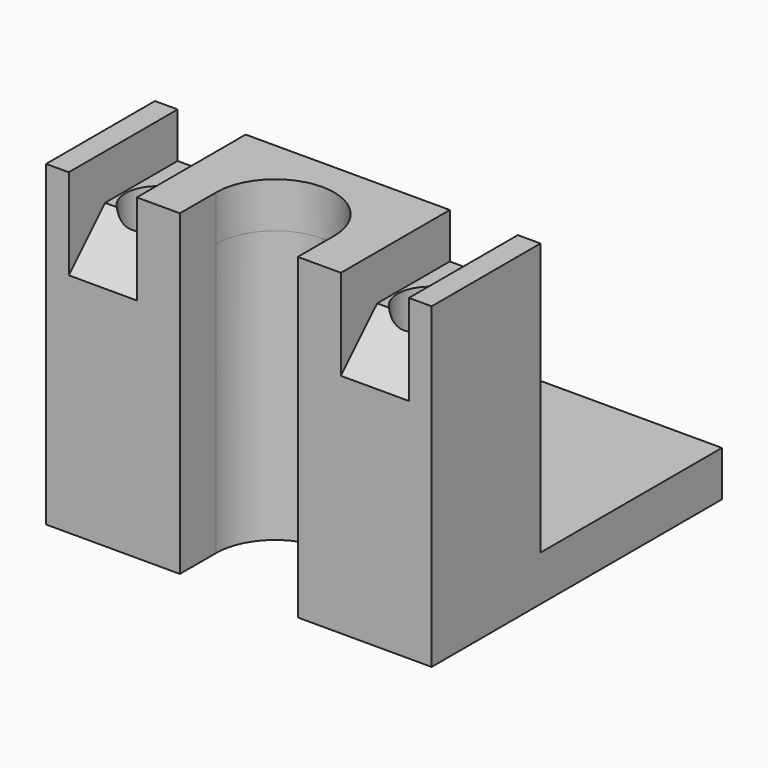
from build123d import *

# Parameters (mm, degrees)
F1_DEPTH    = 12
F0_W        = 8.5
F0_H        = 10
F2_DEPTH    = 2
F4_D        = 2.8
F6_W        = 1
F6_H        = 6
F7_DEPTH    = 2
F8_T1_DEPTH = 3
F8_T3_DEPTH = 3


# Not quite as in the source:
# - a fillet or chamfer that OpenCascade refuses, or shapes differently, is made with other operations: its cross-section is extruded or revolved along the edge and cut away or added


with BuildPart() as f1:
    # F0 (on Top) → F1 (new body)
    with BuildSketch(Plane.XY):
        with BuildLine():
            Line((0, 2), (0, 0))
            Line((0, 0), (5.9, 0))
            Line((5.9, 0), (5.9, 6))
            Line((5.9, 6), (-2.6, 6))
            Line((-2.6, 6), (-2.6, 4.6))
            ThreePointArc((-2.6, 4.6), (-0.7615223689, 3.8384776311), (0, 2))
        make_face()
    extrude(amount=F1_DEPTH)

    # F0 (on Top) → F2 (join)
    with BuildSketch(Plane.XY):
        with Locations((1.65, 11)):
            Rectangle(F0_W, F0_H)
    extrude(amount=F2_DEPTH)

    # F4 (through all)
    with Locations(Plane.XY.offset(12)):
        with Locations((3.4, 3)):
            Hole(F4_D / 2)

    # F5: F1 across face


with BuildPart() as f1_1:
    add(f1.part)
    add(f1.part.mirror(Plane(origin=(-2.6, 8.397826087, 3.2826086957), x_dir=(0, -1, 0), z_dir=(-1, 0, 0))))

    # F6 (on face) → F7 (join)
    with BuildSketch(Plane.XY.offset(12)):
        with Locations((-10.6, 3)):
            Rectangle(F6_W, F6_H)
        with BuildLine():
            Line((1.9, 6), (-7.1, 6))
            Line((-7.1, 6), (-7.1, 0))
            Line((-7.1, 0), (-5.2, 0))
            Line((-5.2, 0), (-5.2, 2))
            ThreePointArc((-5.2, 2), (-2.6, 4.6), (0, 2))
            Line((0, 2), (0, 0))
            Line((0, 0), (1.9, 0))
            Line((1.9, 0), (1.9, 6))
        make_face()
        with Locations((5.4, 3)):
            Rectangle(F6_W, F6_H)
    extrude(amount=F7_DEPTH)

    # F8: chamfer of 2 on 2 edges, made by hand

    # F8_s2 → F8_t1 (cut)
    with BuildSketch(Plane.YZ.offset(-10.1)):
        Polygon((2, 12), (0, 10), (0, 12), align=None)
    extrude(amount=F8_T1_DEPTH, mode=Mode.SUBTRACT)

    # F8_s4 → F8_t3 (cut)
    with BuildSketch(Plane.YZ.offset(1.9)):
        Polygon((2, 12), (0, 10), (0, 12), align=None)
    extrude(amount=F8_T3_DEPTH, mode=Mode.SUBTRACT)


solid = f1_1.part
